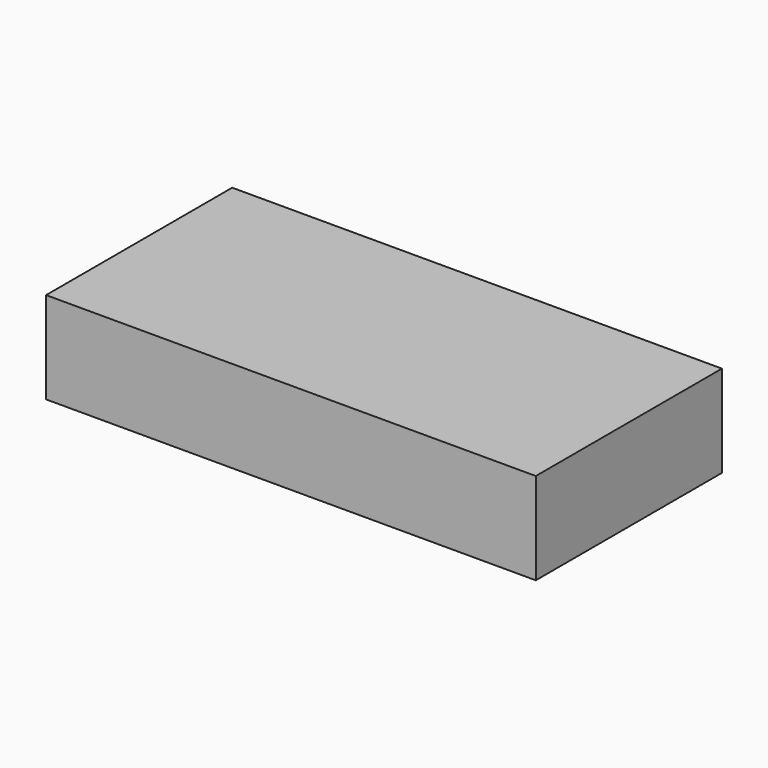
from build123d import *

# Parameters (mm, degrees)
F0_W     = 101.6
F0_H     = 48.26
F1_DEPTH = 19.05


# Not quite as in the source:
# - a feature of the source that left no trace in its solid (it failed there, or was rolled back) is left out


with BuildPart() as f1:
    # F0 (on Top) → F1 (new body)
    with BuildSketch(Plane.XY):
        with Locations((50.8, 24.13)):
            Rectangle(F0_W, F0_H)
    extrude(amount=F1_DEPTH)


solid = f1.part
